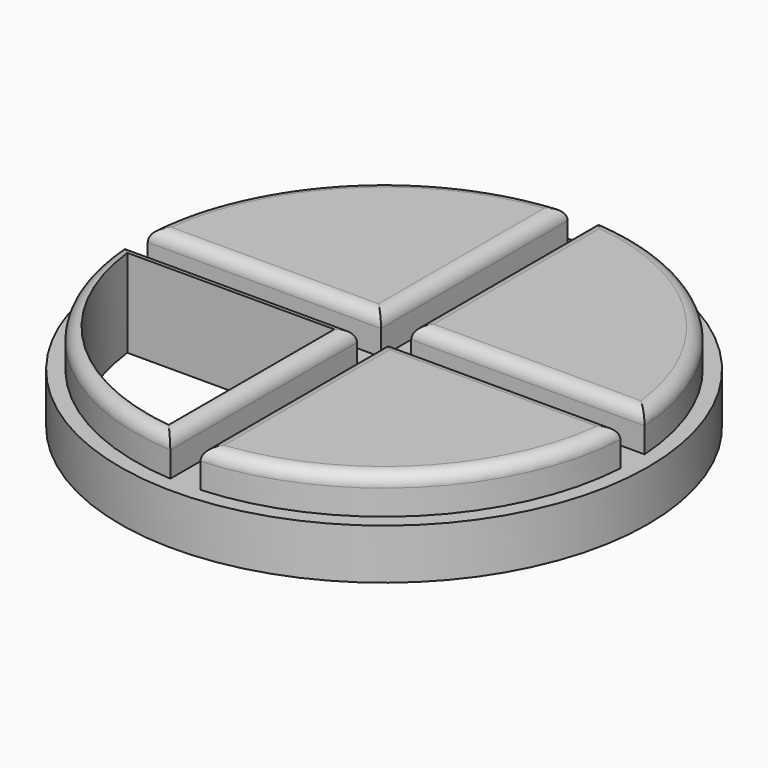
from build123d import *

# Parameters (mm, degrees)
F0_R     = 10.5
F1_DEPTH = 2
F3_DEPTH = 1.5
F4_R     = 0.5
F5_DEPTH = 25


with BuildPart() as f1:
    # F0 (on Top) → F1 (new body)
    with BuildSketch(Plane.XY):
        Circle(F0_R)
    extrude(amount=F1_DEPTH)

    # F2 (on face) → F3 (join)
    with BuildSketch(Plane.XY.offset(2)):
        with BuildLine():
            ThreePointArc((-9.8818014552, -0.6), (-7.0003571337, -7.0003571337), (-0.6, -9.8818014552))
            Line((-0.6, -9.8818014552), (-0.6, -0.6))
            Line((-0.6, -0.6), (-9.8818014552, -0.6))
        make_face()
        with BuildLine():
            Line((-0.6, 0.6), (-0.6, 9.8818014552))
            ThreePointArc((-0.6, 9.8818014552), (-7.0003571337, 7.0003571337), (-9.8818014552, 0.6))
            Line((-9.8818014552, 0.6), (-0.6, 0.6))
        make_face()
        with BuildLine():
            Line((0.6, 0.6), (9.8818014552, 0.6))
            ThreePointArc((9.8818014552, 0.6), (7.0003571337, 7.0003571337), (0.6, 9.8818014552))
            Line((0.6, 9.8818014552), (0.6, 0.6))
        make_face()
        with BuildLine():
            ThreePointArc((0.6, -9.8818014552), (7.0003571337, -7.0003571337), (9.8818014552, -0.6))
            Line((9.8818014552, -0.6), (0.6, -0.6))
            Line((0.6, -0.6), (0.6, -9.8818014552))
        make_face()
    extrude(amount=F3_DEPTH)

    # F4
    f4_edges = [f1.edges().sort_by_distance(p)[0] for p in [
        (-7.000357, -7.000357, 3.5),
        (-0.6, -5.240901, 3.5),
        (-5.240901, -0.6, 3.5),
        (-5.240901, 0.6, 3.5),
        (-0.6, 5.240901, 3.5),
        (5.240901, 0.6, 3.5),
        (0.6, 5.240901, 3.5),
        (5.240901, -0.6, 3.5),
        (0.6, -5.240901, 3.5),
        (7.000357, 7.000357, 3.5),
        (7.000357, -7.000357, 3.5),
        (-7.000357, 7.000357, 3.5),
    ]]
    fillet(f4_edges, radius=F4_R)

    # F5 (cut): a face of the model
    f5_faces = [f1.faces().sort_by_distance(p)[0] for p in [
        (-4.4718926095, -4.4718926095, 3.5),
    ]]
    extrude(f5_faces, amount=-F5_DEPTH, mode=Mode.SUBTRACT)


solid = f1.part
